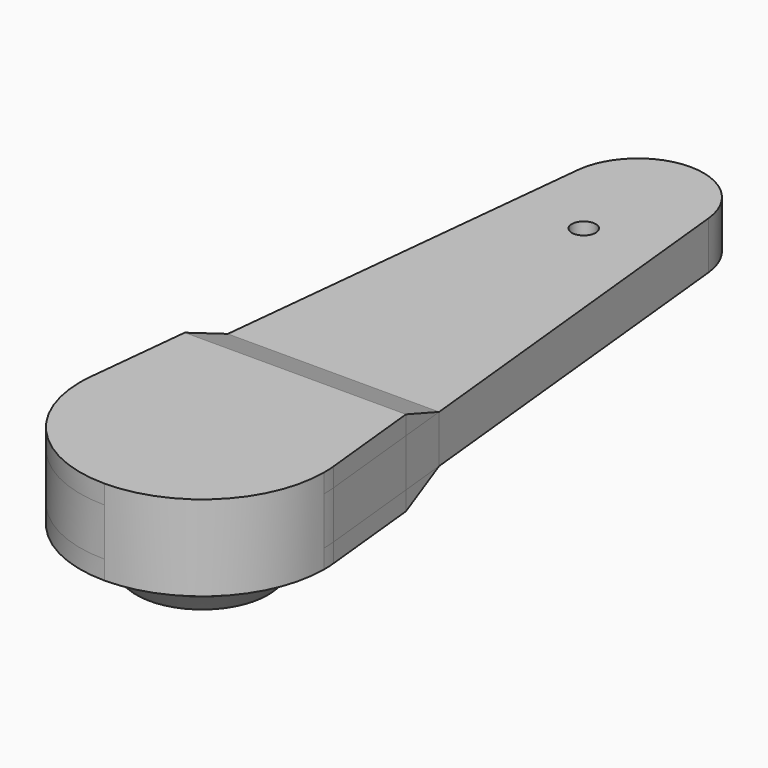
from build123d import *

# Parameters (mm, degrees)
F1_DEPTH  = 1.27
F2_W      = 12.7
F2_H      = 1.0033
F3_DEPTH  = 6.5
F5_DEPTH  = 4.5476
F6_R      = 4.7625
F7_DEPTH  = 2.1844
F8_SIZE   = 1.27
F9_R      = 2.921
F10_DEPTH = 5.08
F11_R     = 0.635
F12_DEPTH = 25.4


# Not quite as in the source:
# - after a boolean that leaves OpenCascade's solid faulty, fix() repairs it


with BuildPart() as f1:
    # F0 (on Top) → F1 (new body, symmetric)
    with BuildSketch(Plane.XY):
        with BuildLine():
            ThreePointArc((-6.465126425, 0.6724137931), (-0.3366587573, -6.4912757514), (6.5, 0))
            ThreePointArc((6.5, 0), (6.4912757514, 0.3366587573), (6.465126425, 0.6724137931))
            ThreePointArc((6.465126425, 0.6724137931), (0, 6.5), (-6.465126425, 0.6724137931))
        make_face()
        with BuildLine():
            ThreePointArc((-6.465126425, 0.6724137931), (0, 6.5), (6.465126425, 0.6724137931))
            Line((6.465126425, 0.6724137931), (3.4812219211, 29.3620689655))
            ThreePointArc((3.4812219211, 29.3620689655), (3.4953023277, 29.1812777924), (3.5, 29))
            ThreePointArc((3.5, 29), (-0.1812777924, 25.5046976723), (-3.4812219211, 29.3620689655))
            Line((-3.4812219211, 29.3620689655), (-6.465126425, 0.6724137931))
        make_face()
        with BuildLine():
            ThreePointArc((3.5, 29), (3.4953023277, 29.1812777924), (3.4812219211, 29.3620689655))
            ThreePointArc((3.4812219211, 29.3620689655), (0, 32.5), (-3.4812219211, 29.3620689655))
            ThreePointArc((-3.4812219211, 29.3620689655), (-0.1812777924, 25.5046976723), (3.5, 29))
        make_face()
    extrude(amount=F1_DEPTH, both=True)

    # F2 (on Right) → F3 (join, symmetric)
    with BuildSketch(Plane.YZ):
        with Locations((-0.15, -1.77165)):
            Rectangle(F2_W, F2_H)
        with Locations((-0.15, 1.77165)):
            Rectangle(F2_W, F2_H)
        Polygon((8.74, 1.27), (6.2, 2.2733), (6.2, 1.27), align=None)
        Polygon((8.74, -1.27), (6.2, -1.27), (6.2, -2.2733), align=None)
    extrude(amount=F3_DEPTH, both=True)

    # F4 (on face) → F5 (cut, through all)
    with BuildSketch(Plane.XY.offset(2.2733)):
        Polygon((5.6260467402, 8.74), (5.8902227087, 6.2), (6.5, 6.2), (6.5, 8.74), align=None)
        with BuildLine():
            Line((6.5, 6.2), (5.8902227087, 6.2))
            Line((5.8902227087, 6.2), (6.465126425, 0.6724137931))
            ThreePointArc((6.465126425, 0.6724137931), (6.4912757514, 0.3366587573), (6.5, 0))
            Line((6.5, 0), (6.5, 6.2))
        make_face()
        with BuildLine():
            ThreePointArc((6.5, 0), (4.5961940777, -4.5961940777), (0, -6.5))
            Line((0, -6.5), (6.5, -6.5))
            Line((6.5, -6.5), (6.5, 0))
        make_face()
        with BuildLine():
            ThreePointArc((0, -6.5), (-4.5961940777, -4.5961940777), (-6.5, 0))
            Line((-6.5, 0), (-6.5, -6.5))
            Line((-6.5, -6.5), (0, -6.5))
        make_face()
        Polygon((-6.5, 6.2), (-5.8902227087, 6.2), (-5.6260467402, 8.74), (-6.5, 8.74), align=None)
        with BuildLine():
            ThreePointArc((-6.5, 0), (-6.4912757514, 0.3366587573), (-6.465126425, 0.6724137931))
            Line((-6.465126425, 0.6724137931), (-5.8902227087, 6.2))
            Line((-5.8902227087, 6.2), (-6.5, 6.2))
            Line((-6.5, 6.2), (-6.5, 0))
        make_face()
    extrude(amount=-F5_DEPTH, mode=Mode.SUBTRACT)

    add(f1.part.fix(), mode=Mode.REPLACE)

    # F6 (on face) → F7 (join)
    with BuildSketch(Plane(origin=(0, 0, -2.2733), x_dir=(1, 0, 0), z_dir=(0, 0, -1))):
        Circle(F6_R)
    extrude(amount=F7_DEPTH)

    # F8
    f8_edges = [f1.edges().sort_by_distance(p)[0] for p in [
        (-4.7625, 0, -4.4577),
    ]]
    chamfer(f8_edges, length=F8_SIZE)

    # F9 (on face) → F10 (cut)
    with BuildSketch(Plane(origin=(0, 0, -4.4577), x_dir=(1, 0, 0), z_dir=(0, 0, -1))):
        Circle(F9_R)
    extrude(amount=-F10_DEPTH, mode=Mode.SUBTRACT)

    add(f1.part.fix(), mode=Mode.REPLACE)

    # F11 (on face) → F12 (cut)
    with BuildSketch(Plane.XY.offset(1.27)):
        with Locations((0, 25.4)):
            Circle(F11_R)
    extrude(amount=-F12_DEPTH, mode=Mode.SUBTRACT)


solid = f1.part
